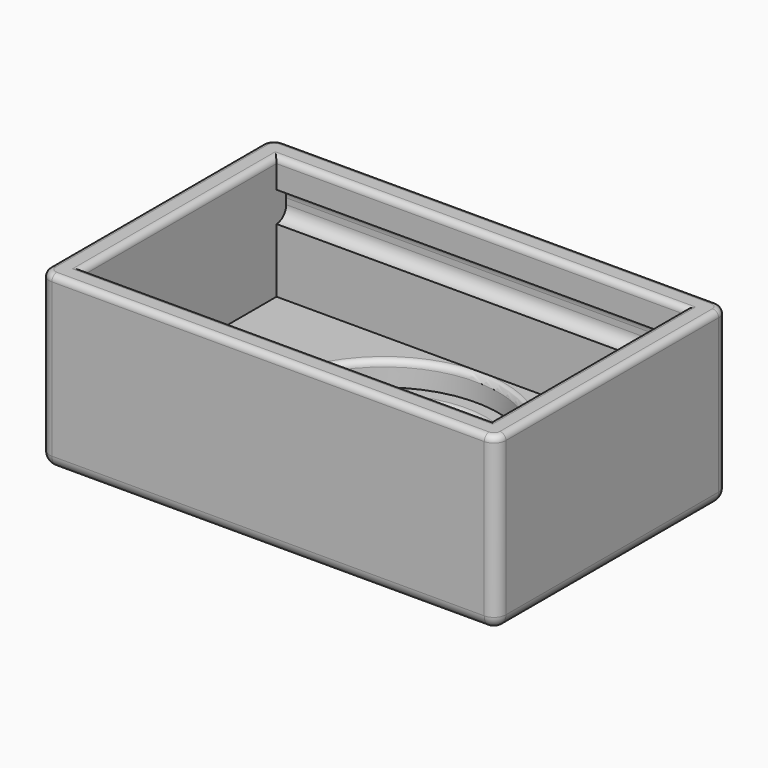
from build123d import *

# Parameters (mm, degrees)
F0_W          = 37.8
F0_H          = 24
F0_W_2        = 33.8
F0_H_2        = 20
F1_DEPTH      = 14.2
F0_R          = 9.5
F2_DEPTH      = 4
F0_R_2        = 8
F3_DEPTH      = 2
F4_W          = 33.8
F4_H          = 2.5
F5_DEPTH      = 1
F7_DEPTH      = 1
F8_R          = 0.49999
F9_R          = 0.99999
F10_T1_DEPTH  = 35.8
F10_T3_DEPTH  = 22
F10_T5_DEPTH  = 13.2
F10_T8_ANGLE  = 90
F10_T10_ANGLE = 90
F10_T12_ANGLE = 90
F10_T14_ANGLE = 90
F10_S17_W     = 1
F10_S17_H     = 1
F10_T18_DEPTH = 1
F10_S23_W     = 1
F10_S23_H     = 1
F10_T24_DEPTH = 1
F10_S29_W     = 1
F10_S29_H     = 1
F10_T30_DEPTH = 1
F10_S35_W     = 1
F10_S35_H     = 1
F10_T36_DEPTH = 1


# Not quite as in the source:
# - a fillet or chamfer that OpenCascade refuses, or shapes differently, is made with other operations: its cross-section is extruded or revolved along the edge and cut away or added
# - a fillet or chamfer is up to 0.001 mm smaller than in the source, because OpenCascade refuses the exact size


with BuildPart() as f1:
    # F0 (on Top) → F1 (new body)
    with BuildSketch(Plane.XY):
        Rectangle(F0_W, F0_H)
        Rectangle(F0_W_2, F0_H_2, mode=Mode.SUBTRACT)
    extrude(amount=F1_DEPTH)

    # F0 (on Top) → F2 (join)
    with BuildSketch(Plane.XY):
        Rectangle(F0_W_2, F0_H_2)
        Circle(F0_R, mode=Mode.SUBTRACT)
    extrude(amount=F2_DEPTH)

    # F0 (on Top) → F3 (join)
    with BuildSketch(Plane.XY):
        Circle(F0_R)
        Circle(F0_R_2, mode=Mode.SUBTRACT)
    extrude(amount=F3_DEPTH)

    # F4 (on face) → F5 (cut)
    with BuildSketch(Plane.XZ.offset(-10)):
        with Locations((0, 10.55)):
            Rectangle(F4_W, F4_H)
    extrude(amount=-F5_DEPTH, mode=Mode.SUBTRACT)

    # F6 (on face) → F7 (cut)
    with BuildSketch(Plane(origin=(0, -10, 0), x_dir=(-1, 0, 0), z_dir=(0, 1, 0))):
        Polygon((-16.9, 9.3), (1.5624057269, 9.3), (16.9, 9.3), (16.9, 11.8), (-16.9, 11.8), align=None)
    extrude(amount=-F7_DEPTH, mode=Mode.SUBTRACT)

    # F8 (radius 0.5 in the source; OpenCascade refuses exactly that, so slightly less here)
    f8_edges = [f1.edges().sort_by_distance(p)[0] for p in [
        (-9.5, 0, 4),
        (-8, 0, 2),
        (0, 10, 14.2),
        (16.9, 0, 14.2),
        (-16.9, 0, 14.2),
        (0, -10, 14.2),
        (0, -12, 14.2),
        (18.9, 0, 14.2),
        (0, 12, 14.2),
        (-18.9, 0, 14.2),
    ]]
    fillet(f8_edges, radius=F8_R)

    # F9 (radius 1 in the source; OpenCascade refuses exactly that, so slightly less here)
    f9_edges = [f1.edges().sort_by_distance(p)[0] for p in [
        (0, 11, 9.3),
        (0, 11, 11.8),
        (0, -11, 9.3),
        (0, -11, 11.8),
    ]]
    fillet(f9_edges, radius=F9_R)

    # F10: fillet of radius 1 on 8 edges, made by hand

    # F10_s2 → F10_t1 (cut)
    with BuildSketch(Plane.YZ.offset(-17.9)):
        with BuildLine():
            ThreePointArc((-12, 1), (-11.7071067812, 0.2928932188), (-11, 0))
            Line((-11, 0), (-12, 0))
            Line((-12, 0), (-12, 1))
        make_face()
        with BuildLine():
            ThreePointArc((12, 1), (11.7071067812, 0.2928932188), (11, 0))
            Line((11, 0), (12, 0))
            Line((12, 0), (12, 1))
        make_face()
    extrude(amount=F10_T1_DEPTH, mode=Mode.SUBTRACT)

    # F10_s4 → F10_t3 (cut)
    with BuildSketch(Plane.XZ.offset(-11)):
        with BuildLine():
            ThreePointArc((-18.9, 1), (-18.6071067812, 0.2928932188), (-17.9, 0))
            Line((-17.9, 0), (-18.9, 0))
            Line((-18.9, 0), (-18.9, 1))
        make_face()
        with BuildLine():
            ThreePointArc((18.9, 1), (18.6071067812, 0.2928932188), (17.9, 0))
            Line((17.9, 0), (18.9, 0))
            Line((18.9, 0), (18.9, 1))
        make_face()
    extrude(amount=F10_T3_DEPTH, mode=Mode.SUBTRACT)

    # F10_s6 → F10_t5 (cut)
    with BuildSketch(Plane.XY.offset(1)):
        with BuildLine():
            ThreePointArc((17.9, -12), (18.6071067812, -11.7071067812), (18.9, -11))
            Line((18.9, -11), (18.9, -12))
            Line((18.9, -12), (17.9, -12))
        make_face()
        with BuildLine():
            ThreePointArc((-17.9, -12), (-18.6071067812, -11.7071067812), (-18.9, -11))
            Line((-18.9, -11), (-18.9, -12))
            Line((-18.9, -12), (-17.9, -12))
        make_face()
        with BuildLine():
            ThreePointArc((18.9, 11), (18.6071067812, 11.7071067812), (17.9, 12))
            Line((17.9, 12), (18.9, 12))
            Line((18.9, 12), (18.9, 11))
        make_face()
        with BuildLine():
            ThreePointArc((-18.9, 11), (-18.6071067812, 11.7071067812), (-17.9, 12))
            Line((-17.9, 12), (-18.9, 12))
            Line((-18.9, 12), (-18.9, 11))
        make_face()
    extrude(amount=F10_T5_DEPTH, mode=Mode.SUBTRACT)

    # F10_s7 → F10_t8 (revolve, cut)
    with BuildSketch(Plane.YZ.offset(-17.9)):
        with BuildLine():
            ThreePointArc((11.50001, 14.2), (11.8535563195, 14.0535563195), (12, 13.70001))
            Line((12, 13.70001), (12, 14.2))
            Line((12, 14.2), (11.50001, 14.2))
        make_face()
    revolve(axis=Axis((-17.9, 11, 14.2), (0, 0, 1)), revolution_arc=F10_T8_ANGLE, mode=Mode.SUBTRACT)

    # F10_s9 → F10_t10 (revolve, cut)
    with BuildSketch(Plane.XZ.offset(-11)):
        with BuildLine():
            ThreePointArc((18.40001, 14.2), (18.7535563195, 14.0535563195), (18.9, 13.70001))
            Line((18.9, 13.70001), (18.9, 14.2))
            Line((18.9, 14.2), (18.40001, 14.2))
        make_face()
    revolve(axis=Axis((17.9, 11, 14.2), (0, 0, 1)), revolution_arc=F10_T10_ANGLE, mode=Mode.SUBTRACT)

    # F10_s11 → F10_t12 (revolve, cut)
    with BuildSketch(Plane.XZ.offset(11)):
        with BuildLine():
            ThreePointArc((-18.40001, 14.2), (-18.7535563195, 14.0535563195), (-18.9, 13.70001))
            Line((-18.9, 13.70001), (-18.9, 14.2))
            Line((-18.9, 14.2), (-18.40001, 14.2))
        make_face()
    revolve(axis=Axis((-17.9, -11, 14.2), (0, 0, 1)), revolution_arc=F10_T12_ANGLE, mode=Mode.SUBTRACT)

    # F10_s13 → F10_t14 (revolve, cut)
    with BuildSketch(Plane.YZ.offset(17.9)):
        with BuildLine():
            ThreePointArc((-11.50001, 14.2), (-11.8535563195, 14.0535563195), (-12, 13.70001))
            Line((-12, 13.70001), (-12, 14.2))
            Line((-12, 14.2), (-11.50001, 14.2))
        make_face()
    revolve(axis=Axis((17.9, -11, 14.2), (0, 0, 1)), revolution_arc=F10_T14_ANGLE, mode=Mode.SUBTRACT)


with BuildPart() as f10_tool16:
    # F10_s17 → F10_t18 (new body)
    with BuildSketch(Plane.XY.offset(1)):
        with Locations((-18.4, -11.5)):
            Rectangle(F10_S17_W, F10_S17_H)
    extrude(amount=-F10_T18_DEPTH)

    # F10_s19 → F10_t20 (revolve, cut)
    with BuildSketch(Plane(origin=(-17.9, -11, 1), x_dir=(0.7071067812, 0.7071067812, 0), z_dir=(-0.7071067812, 0.7071067812, 0))):
        with BuildLine():
            ThreePointArc((0, -1), (1, 0), (0, 1))
            Line((0, 1), (0, -1))
        make_face()
    revolve(axis=Axis((-17.9, -11, 1), (0, 0, -1)), mode=Mode.SUBTRACT)


with BuildPart() as f1_1:
    add(f1.part)

    # F10_t15: cut F10_tool16
    add(f10_tool16.part, mode=Mode.SUBTRACT)


with BuildPart() as f10_tool22:
    # F10_s23 → F10_t24 (new body)
    with BuildSketch(Plane.XY.offset(1)):
        with Locations((18.4, -11.5)):
            Rectangle(F10_S23_W, F10_S23_H)
    extrude(amount=-F10_T24_DEPTH)

    # F10_s25 → F10_t26 (revolve, cut)
    with BuildSketch(Plane(origin=(17.9, -11, 1), x_dir=(-0.7071067812, 0.7071067812, 0), z_dir=(-0.7071067812, -0.7071067812, 0))):
        with BuildLine():
            ThreePointArc((0, -1), (1, 0), (0, 1))
            Line((0, 1), (0, -1))
        make_face()
    revolve(axis=Axis((17.9, -11, 1), (0, 0, -1)), mode=Mode.SUBTRACT)


with BuildPart() as f1_2:
    add(f1_1.part)

    # F10_t21: cut F10_tool22
    add(f10_tool22.part, mode=Mode.SUBTRACT)


with BuildPart() as f10_tool28:
    # F10_s29 → F10_t30 (new body)
    with BuildSketch(Plane.XY.offset(1)):
        with Locations((-18.4, 11.5)):
            Rectangle(F10_S29_W, F10_S29_H)
    extrude(amount=-F10_T30_DEPTH)

    # F10_s31 → F10_t32 (revolve, cut)
    with BuildSketch(Plane(origin=(-17.9, 11, 1), x_dir=(0.7071067812, -0.7071067812, 0), z_dir=(0.7071067812, 0.7071067812, 0))):
        with BuildLine():
            ThreePointArc((0, -1), (1, 0), (0, 1))
            Line((0, 1), (0, -1))
        make_face()
    revolve(axis=Axis((-17.9, 11, 1), (0, 0, -1)), mode=Mode.SUBTRACT)


with BuildPart() as f1_3:
    add(f1_2.part)

    # F10_t27: cut F10_tool28
    add(f10_tool28.part, mode=Mode.SUBTRACT)


with BuildPart() as f10_tool34:
    # F10_s35 → F10_t36 (new body)
    with BuildSketch(Plane.XY.offset(1)):
        with Locations((18.4, 11.5)):
            Rectangle(F10_S35_W, F10_S35_H)
    extrude(amount=-F10_T36_DEPTH)

    # F10_s37 → F10_t38 (revolve, cut)
    with BuildSketch(Plane(origin=(17.9, 11, 1), x_dir=(-0.7071067812, -0.7071067812, 0), z_dir=(0.7071067812, -0.7071067812, 0))):
        with BuildLine():
            ThreePointArc((0, -1), (1, 0), (0, 1))
            Line((0, 1), (0, -1))
        make_face()
    revolve(axis=Axis((17.9, 11, 1), (0, 0, -1)), mode=Mode.SUBTRACT)


with BuildPart() as f1_4:
    add(f1_3.part)

    # F10_t33: cut F10_tool34
    add(f10_tool34.part, mode=Mode.SUBTRACT)


solid = f1_4.part
